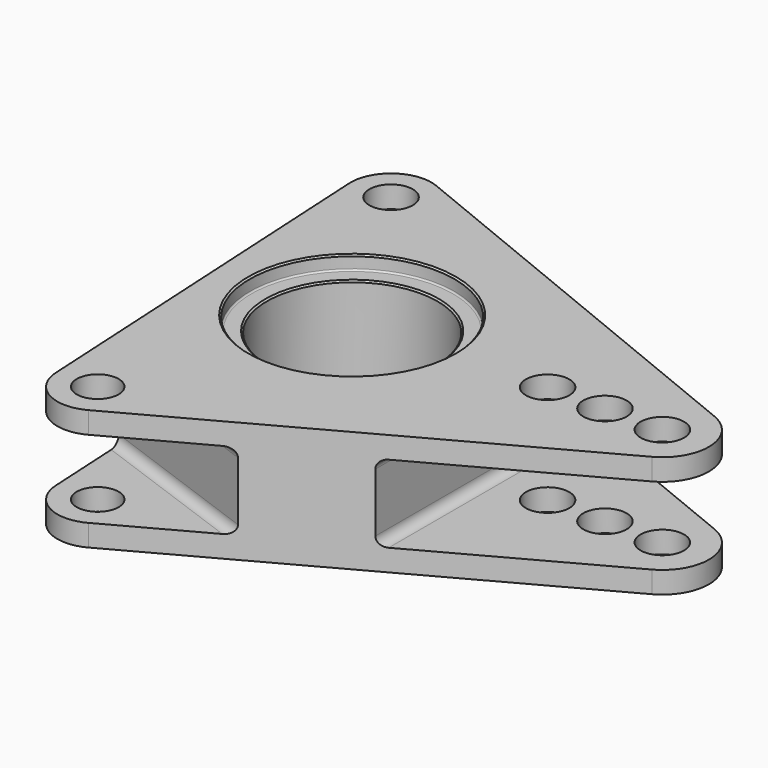
from build123d import *

# Parameters (mm, degrees)
F0_R          = 6.75
F0_R_2        = 33
F0_R_3        = 7
F0_R_4        = 27.48975
F1_DEPTH      = 19.5
F1_DEPTH_BACK = 19.5
F2_START      = 15
F2_DEPTH      = 10
F6_DEPTH      = 12.5
F6_DEPTH_BACK = 12.5
F7_R          = 3
F8_SIZE       = 0.5
F9_R          = 0.5


# Not quite as in the source:
# - a feature names something its author has since deleted; it is built from what else it names


with BuildPart() as f1:
    # F0 (on Top) → F1 (new body, two sides)
    with BuildSketch(Plane.XY) as f1_sk:
        with BuildLine():
            Line((-19.4499833155, -81.9024031138), (107.1556085776, -13.1832191017))
            ThreePointArc((107.1556085776, -13.1832191017), (114.9775485096, 0.8203905436), (105.6729061946, 13.8858969933))
            Line((105.6729061946, 13.8858969933), (-27.583481298, 68.3260953068))
            ThreePointArc((-27.583481298, 68.3260953068), (-40.0371705269, 66.8836794016), (-45.4810708907, 55.5903677578))
            Line((-45.4810708907, 55.5903677578), (-38.6325816401, -71.1782300471))
            ThreePointArc((-38.6325816401, -71.1782300471), (-31.9952103295, -81.8240816881), (-19.4499833155, -81.9024031138))
        make_face()
        with Locations((-25.6515107494, -70.4769465589)):
            Circle(F0_R, mode=Mode.SUBTRACT)
        Circle(F0_R_2, mode=Mode.SUBTRACT)
        with Locations((-32.5, 56.291651246)):
            Circle(F0_R_3, mode=Mode.SUBTRACT)
        with Locations((63, 0)):
            Circle(F0_R_3, mode=Mode.SUBTRACT)
        with Locations((81.5, 0)):
            Circle(F0_R_3, mode=Mode.SUBTRACT)
        with Locations((100, 0)):
            Circle(F0_R_3, mode=Mode.SUBTRACT)
        Circle(F0_R_2)
        Circle(F0_R_4, mode=Mode.SUBTRACT)
    extrude(amount=F1_DEPTH)
    extrude(f1_sk.sketch, amount=-F1_DEPTH_BACK)


with BuildPart() as f2:
    # F0 (on Top) → F2 (new body)
    with BuildSketch(Plane.XY.offset(F2_START)):
        Circle(F0_R_2)
        Circle(F0_R_4, mode=Mode.SUBTRACT)
    extrude(amount=F2_DEPTH)


with BuildPart() as f3_1:
    # F3: instance of F2
    add(f2.part.mirror(Plane.XY))


with BuildPart() as f1_1:
    add(f1.part)

    # F4: cut F2, F3_1
    add(f2.part, mode=Mode.SUBTRACT)
    add(f3_1.part, mode=Mode.SUBTRACT)

    # F5 (on Top) → F6 (cut, two sides)
    with BuildSketch(Plane.XY) as f6_sk:
        Polygon((-66.9979324298, -150.1462552281), (233.1545138204, 12.7709657028), (-82.7719960075, 141.8387137572), (-75.4085285246, 5.5376386383), (45, 75.0555349947), (45, -74.9084380282), (-73.3904532444, -31.8178370259), align=None)
    extrude(amount=-F6_DEPTH, mode=Mode.SUBTRACT)
    extrude(f6_sk.sketch, amount=F6_DEPTH_BACK, mode=Mode.SUBTRACT)

    # F7
    f7_edges = [f1_1.edges().sort_by_distance(p)[0] for p in [
        (45, -4.12355, -12.5),
        (-17.833672, 38.778497, -12.5),
        (-17.833672, 38.778497, 12.5),
        (45, -4.12355, 12.5),
        (-12.985509, -53.803439, 12.5),
        (-12.985509, -53.803439, -12.5),
    ]]
    fillet(f7_edges, radius=F7_R)

    # F8
    f8_edges = [f1_1.edges().sort_by_distance(p)[0] for p in [
        (-27.48975, 0, 15),
        (-27.48975, 0, -15),
        (-33, 0, 19.5),
        (-33, 0, -19.5),
    ]]
    chamfer(f8_edges, length=F8_SIZE)

    # F9
    f9_edges = [f1_1.edges().sort_by_distance(p)[0] for p in [
        (-33, 0, -15),
        (-33, 0, 15),
    ]]
    fillet(f9_edges, radius=F9_R)


solid = f1_1.part
